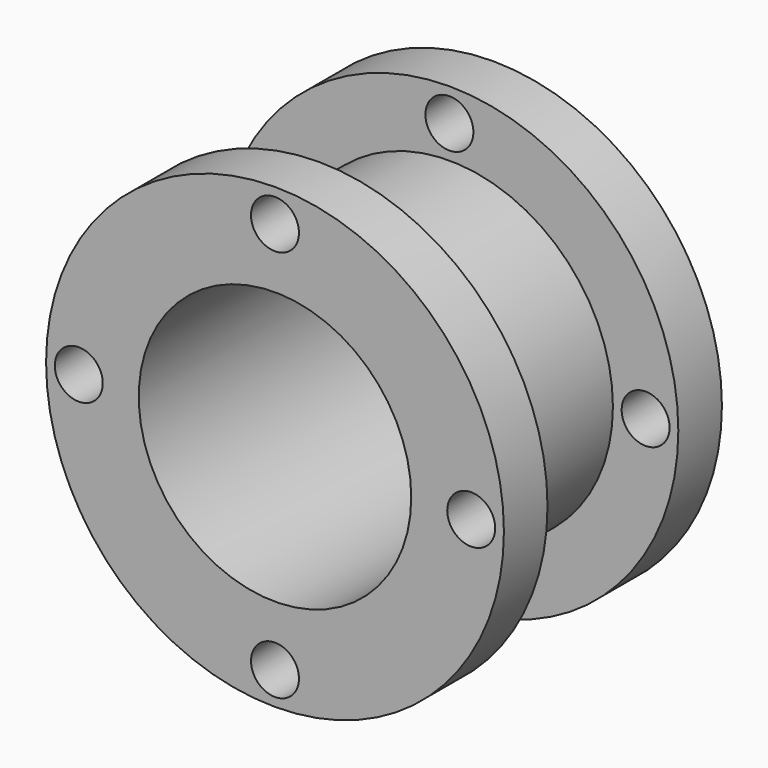
from build123d import *

# Parameters (mm, degrees)
F0_R     = 15
F0_R_2   = 12.5
F1_DEPTH = 25
F0_R_3   = 21
F3_DEPTH = 5
F4_R     = 21
F4_R_2   = 15
F5_DEPTH = 5
F6_D     = 4.4


# Not quite as in the source:
# - the program builds the solid bodies; features that only make, move or delete a surface that nothing else refers to are left out


with BuildPart() as f1:
    # F0 (on Front) → F1 (new body)
    with BuildSketch(Plane.XZ):
        Circle(F0_R)
        Circle(F0_R_2, mode=Mode.SUBTRACT)
    extrude(amount=F1_DEPTH)

    # F0 (on Front) → F3 (join)
    with BuildSketch(Plane.XZ):
        Circle(F0_R_3)
        Circle(F0_R, mode=Mode.SUBTRACT)
    extrude(amount=F3_DEPTH)

    # F4 (on face) → F5 (join)
    with BuildSketch(Plane.XZ.offset(25)):
        Circle(F4_R)
        Circle(F4_R_2, mode=Mode.SUBTRACT)
    extrude(amount=-F5_DEPTH)

    # F6 (through all)
    with Locations(Plane(origin=(0, 0, 0), x_dir=(1, 0, 0), z_dir=(0, 1, 0))):
        with Locations((-18, 0), (0, 18), (18, 0), (0, -18)):
            Hole(F6_D / 2)


solid = f1.part
